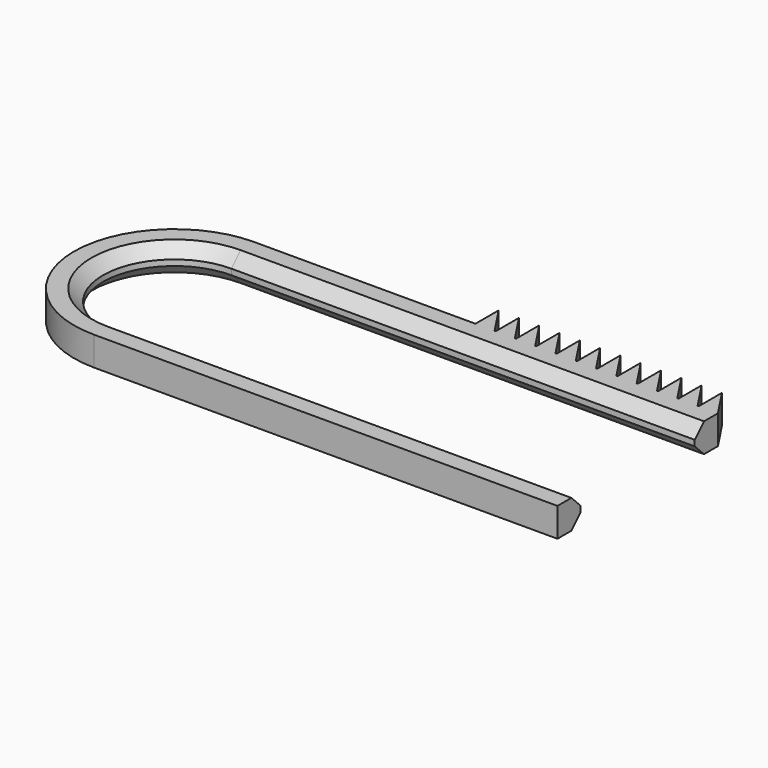
from build123d import *

# Parameters (mm, degrees)
F1_DEPTH = 5
F2_SIZE  = 2


# Not quite as in the source:
# - a feature names something its author has since deleted; it is built from what else it names


with BuildPart() as f1:
    # F0 (on Top) → F1 (new body)
    with BuildSketch(Plane.XY):
        with BuildLine():
            ThreePointArc((-64.1, -12.3136591911), (-76.4136591911, 0), (-64.1, 12.3136591911))
            Line((-64.1, 12.3136591911), (0, 12.3136591911))
            Line((0, 12.3136591911), (15.9, 12.3136591911))
            Line((15.9, 12.3136591911), (15.9, 17.3136591911))
            Line((15.9, 17.3136591911), (12.5920902938, 17.3136591911))
            Line((12.5920902938, 17.3136591911), (12.395, 17.3136591911))
            Line((12.395, 17.3136591911), (9.0870902938, 17.3136591911))
            Line((9.0870902938, 17.3136591911), (8.89, 17.3136591911))
            Line((8.89, 17.3136591911), (5.5820902938, 17.3136591911))
            Line((5.5820902938, 17.3136591911), (5.3854580642, 17.3136591911))
            Line((5.3854580642, 17.3136591911), (2.077548358, 17.3136591911))
            Line((2.077548358, 17.3136591911), (1.8804580642, 17.3136591911))
            Line((1.8804580642, 17.3136591911), (0, 17.3136591911))
            Line((0, 17.3136591911), (-1.427451642, 17.3136591911))
            Line((-1.427451642, 17.3136591911), (-1.6245419358, 17.3136591911))
            Line((-1.6245419358, 17.3136591911), (-4.932451642, 17.3136591911))
            Line((-4.932451642, 17.3136591911), (-5.1295419358, 17.3136591911))
            Line((-5.1295419358, 17.3136591911), (-8.437451642, 17.3136591911))
            Line((-8.437451642, 17.3136591911), (-8.6340838715, 17.3136591911))
            Line((-8.6340838715, 17.3136591911), (-11.9419935778, 17.3136591911))
            Line((-11.9419935778, 17.3136591911), (-12.1390838715, 17.3136591911))
            Line((-12.1390838715, 17.3136591911), (-15.4469935778, 17.3136591911))
            Line((-15.4469935778, 17.3136591911), (-15.6440838715, 17.3136591911))
            Line((-15.6440838715, 17.3136591911), (-18.9519935778, 17.3136591911))
            Line((-18.9519935778, 17.3136591911), (-19.1490838715, 17.3136591911))
            Line((-19.1490838715, 17.3136591911), (-22.4569935778, 17.3136591911))
            Line((-22.4569935778, 17.3136591911), (-22.6536258073, 17.3136591911))
            Line((-22.6536258073, 17.3136591911), (-25.9615355136, 17.3136591911))
            Line((-25.9615355136, 17.3136591911), (-64.1, 17.3136591911))
            ThreePointArc((-64.1, 17.3136591911), (-81.4136591911, 0), (-64.1, -17.3136591911))
            Line((-64.1, -17.3136591911), (0, -17.3136591911))
            Line((0, -17.3136591911), (15.9, -17.3136591911))
            Line((15.9, -17.3136591911), (15.9, -12.3136591911))
            Line((15.9, -12.3136591911), (0, -12.3136591911))
            Line((0, -12.3136591911), (-64.1, -12.3136591911))
        make_face()
        Polygon((12.5920902938, 17.3136591911), (15.9, 17.3136591911), (12.5920902938, 22.3136591911), align=None)
        Polygon((9.0870902938, 17.3136591911), (12.395, 17.3136591911), (9.0870902938, 22.3136591911), align=None)
        Polygon((5.5820902938, 17.3136591911), (8.89, 17.3136591911), (5.5820902938, 22.3136591911), align=None)
        Polygon((2.077548358, 17.3136591911), (5.3854580642, 17.3136591911), (2.077548358, 22.3136591911), align=None)
        Polygon((0, 17.3136591911), (1.8804580642, 17.3136591911), (-1.427451642, 22.3136591911), (-1.427451642, 17.3136591911), align=None)
        Polygon((-4.932451642, 17.3136591911), (-1.6245419358, 17.3136591911), (-4.932451642, 22.3136591911), align=None)
        Polygon((-8.437451642, 17.3136591911), (-5.1295419358, 17.3136591911), (-8.437451642, 22.3136591911), align=None)
        Polygon((-11.9419935778, 22.3136591911), (-11.9419935778, 17.3136591911), (-8.6340838715, 17.3136591911), align=None)
        Polygon((-15.4469935778, 22.3136591911), (-15.4469935778, 17.3136591911), (-12.1390838715, 17.3136591911), align=None)
        Polygon((-18.9519935778, 22.3136591911), (-18.9519935778, 17.3136591911), (-15.6440838715, 17.3136591911), align=None)
        Polygon((-22.4569935778, 22.3136591911), (-22.4569935778, 17.3136591911), (-19.1490838715, 17.3136591911), align=None)
        Polygon((-25.9615355136, 22.3136591911), (-25.9615355136, 17.3136591911), (-22.6536258073, 17.3136591911), align=None)
    extrude(amount=F1_DEPTH)

    # F2
    f2_edges = [f1.edges().sort_by_distance(p)[0] for p in [
        (-76.413659, 0, 5),
        (-76.413659, 0, 0),
    ]]
    chamfer(f2_edges, length=F2_SIZE)


solid = f1.part
